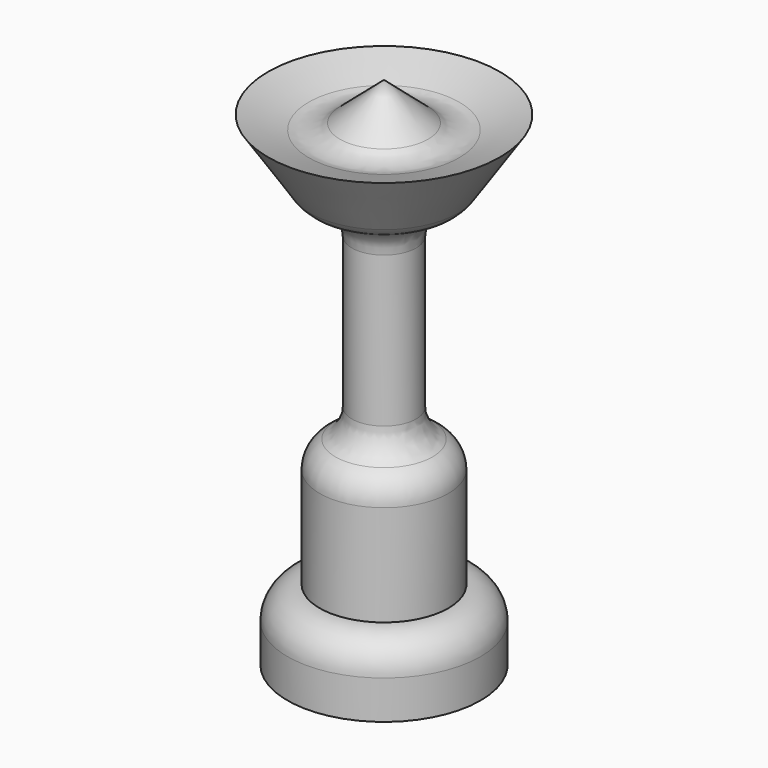
from build123d import *

# Parameters (mm, degrees)
F2_R = 4.8284271247
F3_R = 4.99999
F4_R = 5
F5_R = 5
F6_R = 5
F7_R = 5


# Not quite as in the source:
# - a fillet or chamfer is up to 0.001 mm smaller than in the source, because OpenCascade refuses the exact size


with BuildPart() as f1:
    # F0 (on Front) → F1 (revolve)
    with BuildSketch(Plane.XZ):
        Polygon((0, 55.4385791123), (0, -7.8231290636), (15, -7.8231290636), (15, 3.1768709364), (10, 3.1768709364), (10, 23.6928891391), (5, 23.6928891391), (5, 55.4385791123), (10, 55.4385791123), (18, 67.4385791123), (9, 64.4385791123), (0, 72.1768709364), (0, 61.4385791123), align=None)
    revolve(axis=Axis((0, 0, 26.8077250243), (0, 0, 1)))

    # F2
    f2_edges = [f1.edges().sort_by_distance(p)[0] for p in [
        (-10, 0, 23.692889),
    ]]
    fillet(f2_edges, radius=F2_R)

    # F3 (radius 5 in the source; OpenCascade refuses exactly that, so slightly less here)
    f3_edges = [f1.edges().sort_by_distance(p)[0] for p in [
        (-15, 0, 3.176871),
    ]]
    fillet(f3_edges, radius=F3_R)

    # F4
    f4_edges = [f1.edges().sort_by_distance(p)[0] for p in [
        (-5, 0, 23.692889),
    ]]
    fillet(f4_edges, radius=F4_R)

    # F5
    f5_edges = [f1.edges().sort_by_distance(p)[0] for p in [
        (-10, 0, 55.438579),
    ]]
    fillet(f5_edges, radius=F5_R)

    # F6
    f6_edges = [f1.edges().sort_by_distance(p)[0] for p in [
        (-9, 0, 64.438579),
    ]]
    fillet(f6_edges, radius=F6_R)

    # F7
    f7_edges = [f1.edges().sort_by_distance(p)[0] for p in [
        (-5, 0, 55.438579),
    ]]
    fillet(f7_edges, radius=F7_R)


solid = f1.part
